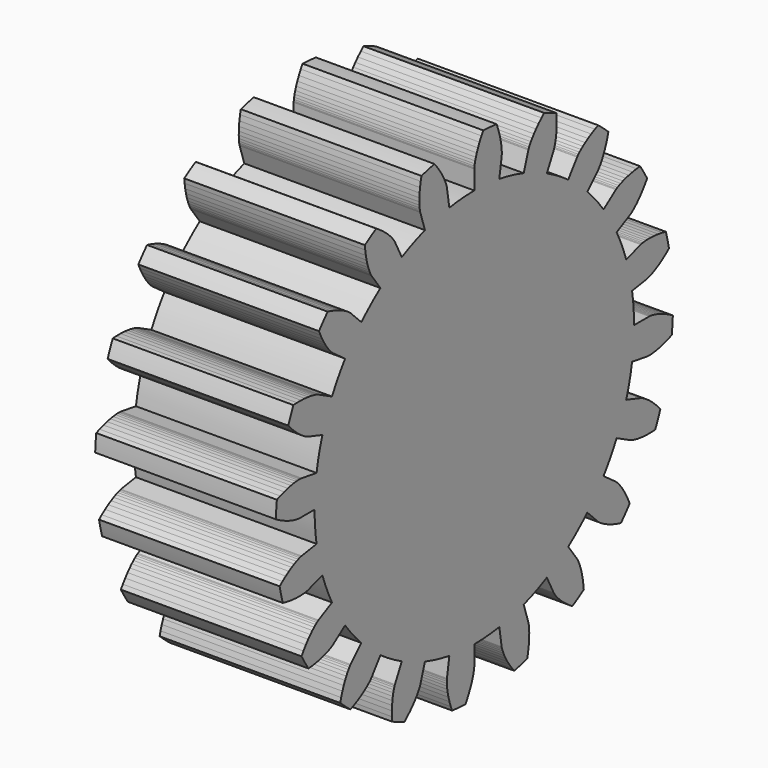
from build123d import *

# Parameters (mm, degrees)
F2_DEPTH = 12.7


# Not quite as in the source:
# - a variable given as a bare number and used for a length is read in inches; the dataset says mm whatever the document's units were


with BuildPart() as f2:
    # F1 (on Right) → F2 (new body)
    with BuildSketch(Plane.YZ):
        with BuildLine():
            ThreePointArc((13.8654281935, -2.1960680843), (13.9949872217, -1.1014293813), (14.0382625, 0))
            ThreePointArc((14.0382625, 0), (13.9949872217, 1.1014293813), (13.8654281935, 2.1960680843))
            ThreePointArc((13.8654281935, 2.1960680843), (13.6503841896, 3.2771672972), (13.3511810281, 4.338061684))
            ThreePointArc((13.3511810281, 4.338061684), (12.9696633958, 5.3722104779), (12.5081834758, 6.3732378078))
            ThreePointArc((12.5081834758, 6.3732378078), (11.9695864452, 7.3349720074), (11.357192934, 8.2514836653))
            ThreePointArc((11.357192934, 8.2514836653), (10.6747785517, 9.1171221826), (9.9265506098, 9.9265506098))
            ThreePointArc((9.9265506098, 9.9265506098), (9.1171221826, 10.6747785517), (8.2514836653, 11.357192934))
            ThreePointArc((8.2514836653, 11.357192934), (7.3349720074, 11.9695864452), (6.3732378078, 12.5081834758))
            ThreePointArc((6.3732378078, 12.5081834758), (5.3722104779, 12.9696633958), (4.338061684, 13.3511810281))
            ThreePointArc((4.338061684, 13.3511810281), (3.2771672972, 13.6503841896), (2.1960680843, 13.8654281935))
            ThreePointArc((2.1960680843, 13.8654281935), (1.1014293813, 13.9949872217), (0, 14.0382625))
            ThreePointArc((0, 14.0382625), (-1.1014293813, 13.9949872217), (-2.1960680843, 13.8654281935))
            ThreePointArc((-2.1960680843, 13.8654281935), (-3.2771672972, 13.6503841896), (-4.338061684, 13.3511810281))
            ThreePointArc((-4.338061684, 13.3511810281), (-5.3722104779, 12.9696633958), (-6.3732378078, 12.5081834758))
            ThreePointArc((-6.3732378078, 12.5081834758), (-7.3349720074, 11.9695864452), (-8.2514836653, 11.357192934))
            ThreePointArc((-8.2514836653, 11.357192934), (-9.1171221826, 10.6747785517), (-9.9265506098, 9.9265506098))
            ThreePointArc((-9.9265506098, 9.9265506098), (-10.6747785517, 9.1171221826), (-11.357192934, 8.2514836653))
            ThreePointArc((-11.357192934, 8.2514836653), (-11.9695864452, 7.3349720074), (-12.5081834758, 6.3732378078))
            ThreePointArc((-12.5081834758, 6.3732378078), (-12.9696633958, 5.3722104779), (-13.3511810281, 4.338061684))
            ThreePointArc((-13.3511810281, 4.338061684), (-13.6503841896, 3.2771672972), (-13.8654281935, 2.1960680843))
            ThreePointArc((-13.8654281935, 2.1960680843), (-13.9949872217, 1.1014293813), (-14.0382625, 0))
            ThreePointArc((-14.0382625, 0), (-13.9949872217, -1.1014293813), (-13.8654281935, -2.1960680843))
            ThreePointArc((-13.8654281935, -2.1960680843), (-13.6503841896, -3.2771672972), (-13.3511810281, -4.338061684))
            ThreePointArc((-13.3511810281, -4.338061684), (-12.9696633958, -5.3722104779), (-12.5081834758, -6.3732378078))
            ThreePointArc((-12.5081834758, -6.3732378078), (-11.9695864452, -7.3349720074), (-11.357192934, -8.2514836653))
            ThreePointArc((-11.357192934, -8.2514836653), (-10.6747785517, -9.1171221826), (-9.9265506098, -9.9265506098))
            ThreePointArc((-9.9265506098, -9.9265506098), (-9.1171221826, -10.6747785517), (-8.2514836653, -11.357192934))
            ThreePointArc((-8.2514836653, -11.357192934), (-7.3349720074, -11.9695864452), (-6.3732378078, -12.5081834758))
            ThreePointArc((-6.3732378078, -12.5081834758), (-5.3722104779, -12.9696633958), (-4.338061684, -13.3511810281))
            ThreePointArc((-4.338061684, -13.3511810281), (-3.2771672972, -13.6503841896), (-2.1960680843, -13.8654281935))
            ThreePointArc((-2.1960680843, -13.8654281935), (-1.1014293813, -13.9949872217), (0, -14.0382625))
            ThreePointArc((0, -14.0382625), (1.1014293813, -13.9949872217), (2.1960680843, -13.8654281935))
            ThreePointArc((2.1960680843, -13.8654281935), (3.2771672972, -13.6503841896), (4.338061684, -13.3511810281))
            ThreePointArc((4.338061684, -13.3511810281), (5.3722104779, -12.9696633958), (6.3732378078, -12.5081834758))
            ThreePointArc((6.3732378078, -12.5081834758), (7.3349720074, -11.9695864452), (8.2514836653, -11.357192934))
            ThreePointArc((8.2514836653, -11.357192934), (9.1171221826, -10.6747785517), (9.9265506098, -9.9265506098))
            ThreePointArc((9.9265506098, -9.9265506098), (10.6747785517, -9.1171221826), (11.357192934, -8.2514836653))
            ThreePointArc((11.357192934, -8.2514836653), (11.9695864452, -7.3349720074), (12.5081834758, -6.3732378078))
            ThreePointArc((12.5081834758, -6.3732378078), (12.9696633958, -5.3722104779), (13.3511810281, -4.338061684))
            ThreePointArc((13.3511810281, -4.338061684), (13.6503841896, -3.2771672972), (13.8654281935, -2.1960680843))
        make_face()
        with BuildLine():
            Line((-14.6171145636, -4.7493884238), (-13.3511810281, -4.338061684))
            ThreePointArc((-13.3511810281, -4.338061684), (-13.6503841896, -3.2771672972), (-13.8654281935, -2.1960680843))
            Line((-13.8654281935, -2.1960680843), (-15.180121665, -2.404295074))
            Line((-15.180121665, -2.404295074), (-15.1989848071, -2.4079309004))
            Line((-15.1989848071, -2.4079309004), (-15.2550320002, -2.4213414721))
            Line((-15.2550320002, -2.4213414721), (-15.3472398712, -2.4482306459))
            Line((-15.3472398712, -2.4482306459), (-15.474308977, -2.4922197725))
            Line((-15.474308977, -2.4922197725), (-15.6346697243, -2.5568294258))
            Line((-15.6346697243, -2.5568294258), (-15.8264894224, -2.6454615286))
            Line((-15.8264894224, -2.6454615286), (-16.0476804424, -2.7613819428))
            Line((-16.0476804424, -2.7613819428), (-16.2959094551, -2.9077035901))
            Line((-16.2959094551, -2.9077035901), (-16.5686077133, -3.0873701663))
            Line((-16.5686077133, -3.0873701663), (-16.8629823421, -3.3031405114))
            Line((-16.8629823421, -3.3031405114), (-17.1077308908, -3.5020636798))
            ThreePointArc((-17.1077308908, -3.5020636798), (-16.9800097349, -4.0765396663), (-16.8330034779, -4.6463857097))
            Line((-16.8330034779, -4.6463857097), (-16.5246216956, -4.7125140346))
            Line((-16.5246216956, -4.7125140346), (-16.1643742939, -4.771123535))
            Line((-16.1643742939, -4.771123535), (-15.8398314481, -4.807405208))
            Line((-15.8398314481, -4.807405208), (-15.5522291405, -4.8250851369))
            Line((-15.5522291405, -4.8250851369), (-15.3025197318, -4.8279523605))
            Line((-15.3025197318, -4.8279523605), (-15.0913689967, -4.8198398218))
            Line((-15.0913689967, -4.8198398218), (-14.9191543558, -4.8046051886))
            Line((-14.9191543558, -4.8046051886), (-14.7859643079, -4.7861116205))
            Line((-14.7859643079, -4.7861116205), (-14.6915990638, -4.7682085524))
            Line((-14.6915990638, -4.7682085524), (-14.635572377, -4.754712566))
            Line((-14.635572377, -4.754712566), (-14.6171145636, -4.7493884238))
        make_face()
        with BuildLine():
            Line((-12.4340603193, -9.0338736178), (-11.357192934, -8.2514836653))
            ThreePointArc((-11.357192934, -8.2514836653), (-11.9695864452, -7.3349720074), (-12.5081834758, -6.3732378078))
            Line((-12.5081834758, -6.3732378078), (-13.6941855903, -6.9775360683))
            Line((-13.6941855903, -6.9775360683), (-13.7110019723, -6.9868229763))
            Line((-13.7110019723, -6.9868229763), (-13.760161926, -7.016896723))
            Line((-13.760161926, -7.016896723), (-13.8395476109, -7.0709636461))
            Line((-13.8395476109, -7.0709636461), (-13.9468041243, -7.1520663048))
            Line((-13.9468041243, -7.1520663048), (-14.0793507771, -7.2630679327))
            Line((-14.0793507771, -7.2630679327), (-14.234393325, -7.4066376182))
            Line((-14.234393325, -7.4066376182), (-14.4089371079, -7.5852362677))
            Line((-14.4089371079, -7.5852362677), (-14.5998010523, -7.8011034073))
            Line((-14.5998010523, -7.8011034073), (-14.8036324824, -8.0562448714))
            Line((-14.8036324824, -8.0562448714), (-15.0169226878, -8.3524214272))
            Line((-15.0169226878, -8.3524214272), (-15.1882217503, -8.6172400636))
            ThreePointArc((-15.1882217503, -8.6172400636), (-14.88922887, -9.1241311864), (-14.5733254998, -9.6206595475))
            Line((-14.5733254998, -9.6206595475), (-14.25960222, -9.5882561103))
            Line((-14.25960222, -9.5882561103), (-13.8988752495, -9.5326744883))
            Line((-13.8988752495, -9.5326744883), (-13.5790050076, -9.466891155))
            Line((-13.5790050076, -9.466891155), (-13.3000155603, -9.3948317659))
            Line((-13.3000155603, -9.3948317659), (-13.0616417792, -9.3203942067))
            Line((-13.0616417792, -9.3203942067), (-12.863332409, -9.2474295583))
            Line((-12.863332409, -9.2474295583), (-12.7042543131, -9.1797233104))
            Line((-12.7042543131, -9.1797233104), (-12.583297877, -9.1209768938))
            Line((-12.583297877, -9.1209768938), (-12.4990835491, -9.0747896001))
            Line((-12.4990835491, -9.0747896001), (-12.4499694926, -9.0446409559))
            Line((-12.4499694926, -9.0446409559), (-12.4340603193, -9.0338736178))
        make_face()
        with BuildLine():
            Line((-9.0338736178, -12.4340603193), (-8.2514836653, -11.357192934))
            ThreePointArc((-8.2514836653, -11.357192934), (-9.1171221826, -10.6747785517), (-9.9265506098, -9.9265506098))
            Line((-9.9265506098, -9.9265506098), (-10.867767217, -10.867767217))
            Line((-10.867767217, -10.867767217), (-10.8808907344, -10.8817961392))
            Line((-10.8808907344, -10.8817961392), (-10.9183513298, -10.9255892331))
            Line((-10.9183513298, -10.9255892331), (-10.9771440047, -11.0015414583))
            Line((-10.9771440047, -11.0015414583), (-11.0540889108, -11.1118187557))
            Line((-11.0540889108, -11.1118187557), (-11.1458468793, -11.2583467456))
            Line((-11.1458468793, -11.2583467456), (-11.248935632, -11.4428004126))
            Line((-11.248935632, -11.4428004126), (-11.3597466163, -11.6665948172))
            Line((-11.3597466163, -11.6665948172), (-11.4745623996, -11.9308768694))
            Line((-11.4745623996, -11.9308768694), (-11.5895745611, -12.2365181973))
            Line((-11.5895745611, -12.2365181973), (-11.7009020117, -12.5841091389))
            Line((-11.7009020117, -12.5841091389), (-11.7819836423, -12.8889009502))
            ThreePointArc((-11.7819836423, -12.8889009502), (-11.340986544, -13.2785891743), (-10.8871088834, -13.6531961976))
            Line((-10.8871088834, -13.6531961976), (-10.5987535266, -13.5254328726))
            Line((-10.5987535266, -13.5254328726), (-10.2728574565, -13.3611008446))
            Line((-10.2728574565, -13.3611008446), (-9.9889709465, -13.1996918361))
            Line((-9.9889709465, -13.1996918361), (-9.7459037905, -13.0449468041))
            Line((-9.7459037905, -13.0449468041), (-9.5421993235, -12.900490929))
            Line((-9.5421993235, -12.900490929), (-9.3761432211, -12.7698164591))
            Line((-9.3761432211, -12.7698164591), (-9.2457733426, -12.6562661558))
            Line((-9.2457733426, -12.6562661558), (-9.1488905769, -12.5630173991))
            Line((-9.1488905769, -12.5630173991), (-9.0830706503, -12.4930670139))
            Line((-9.0830706503, -12.4930670139), (-9.0456768502, -12.4492168713))
            Line((-9.0456768502, -12.4492168713), (-9.0338736178, -12.4340603193))
        make_face()
        with BuildLine():
            Line((-4.7493884238, -14.6171145636), (-4.338061684, -13.3511810281))
            ThreePointArc((-4.338061684, -13.3511810281), (-5.3722104779, -12.9696633958), (-6.3732378078, -12.5081834758))
            Line((-6.3732378078, -12.5081834758), (-6.9775360683, -13.6941855903))
            Line((-6.9775360683, -13.6941855903), (-6.9856820997, -13.711583278))
            Line((-6.9856820997, -13.711583278), (-7.0077764328, -13.764808946))
            Line((-7.0077764328, -13.764808946), (-7.040221061, -13.8552117404))
            Line((-7.040221061, -13.8552117404), (-7.0793224564, -13.9838689663))
            Line((-7.0793224564, -13.9838689663), (-7.1213098312, -14.1515801375))
            Line((-7.1213098312, -14.1515801375), (-7.1623537435, -14.358862176))
            Line((-7.1623537435, -14.358862176), (-7.1985849778, -14.6059457801))
            Line((-7.1985849778, -14.6059457801), (-7.2261136314, -14.8927729763))
            Line((-7.2261136314, -14.8927729763), (-7.2410483324, -15.2189958653))
            Line((-7.2410483324, -15.2189958653), (-7.2395155218, -15.5839765695))
            Line((-7.2395155218, -15.5839765695), (-7.2224428854, -15.8989064095))
            ThreePointArc((-7.2224428854, -15.8989064095), (-6.6826094377, -16.1332463365), (-6.1351861945, -16.3492628766))
            Line((-6.1351861945, -16.3492628766), (-5.9004249921, -16.1386460281))
            Line((-5.9004249921, -16.1386460281), (-5.6412608004, -15.881649558))
            Line((-5.6412608004, -15.881649558), (-5.4211468118, -15.6404147126))
            Line((-5.4211468118, -15.6404147126), (-5.237795054, -15.4181315596))
            Line((-5.237795054, -15.4181315596), (-5.0886999135, -15.2177977161))
            Line((-5.0886999135, -15.2177977161), (-4.9711518072, -15.0422047523))
            Line((-4.9711518072, -15.0422047523), (-4.8822516582, -14.8939254884))
            Line((-4.8822516582, -14.8939254884), (-4.8189261231, -14.7753022297))
            Line((-4.8189261231, -14.7753022297), (-4.7779435107, -14.6884359841))
            Line((-4.7779435107, -14.6884359841), (-4.7559303328, -14.6351767006))
            Line((-4.7559303328, -14.6351767006), (-4.7493884238, -14.6171145636))
        make_face()
        with BuildLine():
            Line((0, -15.369343791), (0, -14.0382625))
            ThreePointArc((0, -14.0382625), (-1.1014293813, -13.9949872217), (-2.1960680843, -13.8654281935))
            Line((-2.1960680843, -13.8654281935), (-2.404295074, -15.180121665))
            Line((-2.404295074, -15.180121665), (-2.406666229, -15.1991851114))
            Line((-2.406666229, -15.1991851114), (-2.4112315526, -15.2566332542))
            Line((-2.4112315526, -15.2566332542), (-2.4141522278, -15.3526373623))
            Line((-2.4141522278, -15.3526373623), (-2.4115825954, -15.4870806511))
            Line((-2.4115825954, -15.4870806511), (-2.3996893598, -15.6595582657))
            Line((-2.3996893598, -15.6595582657), (-2.3746707675, -15.8693784656))
            Line((-2.3746707675, -15.8693784656), (-2.3327756863, -16.1155650045))
            Line((-2.3327756863, -16.1155650045), (-2.2703225136, -16.3968607002))
            Line((-2.2703225136, -16.3968607002), (-2.1837178417, -16.711732181))
            Line((-2.1837178417, -16.711732181), (-2.0694748119, -17.0583757934))
            Line((-2.0694748119, -17.0583757934), (-1.9559190973, -17.3526161352))
            ThreePointArc((-1.9559190973, -17.3526161352), (-1.3700919591, -17.4086689403), (-0.7827087346, -17.4449497932))
            Line((-0.7827087346, -17.4449497932), (-0.6245217488, -17.1720960658))
            Line((-0.6245217488, -17.1720960658), (-0.4574582322, -16.8475917587))
            Line((-0.4574582322, -16.8475917587), (-0.3226630559, -16.5501448238))
            Line((-0.3226630559, -16.5501448238), (-0.2169744437, -16.2820821735))
            Line((-0.2169744437, -16.2820821735), (-0.137083101, -16.0454804341))
            Line((-0.137083101, -16.0454804341), (-0.0795494184, -15.8421572392))
            Line((-0.0795494184, -15.8421572392), (-0.0408211648, -15.6736636222))
            Line((-0.0408211648, -15.6736636222), (-0.0172516049, -15.5412775325))
            Line((-0.0172516049, -15.5412775325), (-0.0051179705, -15.4459984999))
            Line((-0.0051179705, -15.4459984999), (-0.0006402179, -15.3885434651))
            Line((-0.0006402179, -15.3885434651), (0, -15.369343791))
        make_face()
        with BuildLine():
            Line((4.7493884238, -14.6171145636), (4.338061684, -13.3511810281))
            ThreePointArc((4.338061684, -13.3511810281), (3.2771672972, -13.6503841896), (2.1960680843, -13.8654281935))
            Line((2.1960680843, -13.8654281935), (2.404295074, -15.180121665))
            Line((2.404295074, -15.180121665), (2.4079309004, -15.1989848071))
            Line((2.4079309004, -15.1989848071), (2.4213414721, -15.2550320002))
            Line((2.4213414721, -15.2550320002), (2.4482306459, -15.3472398712))
            Line((2.4482306459, -15.3472398712), (2.4922197725, -15.474308977))
            Line((2.4922197725, -15.474308977), (2.5568294258, -15.6346697243))
            Line((2.5568294258, -15.6346697243), (2.6454615286, -15.8264894224))
            Line((2.6454615286, -15.8264894224), (2.7613819428, -16.0476804424))
            Line((2.7613819428, -16.0476804424), (2.9077035901, -16.2959094551))
            Line((2.9077035901, -16.2959094551), (3.0873701663, -16.5686077133))
            Line((3.0873701663, -16.5686077133), (3.3031405114, -16.8629823421))
            Line((3.3031405114, -16.8629823421), (3.5020636798, -17.1077308908))
            ThreePointArc((3.5020636798, -17.1077308908), (4.0765396663, -16.9800097349), (4.6463857097, -16.8330034779))
            Line((4.6463857097, -16.8330034779), (4.7125140346, -16.5246216956))
            Line((4.7125140346, -16.5246216956), (4.771123535, -16.1643742939))
            Line((4.771123535, -16.1643742939), (4.807405208, -15.8398314481))
            Line((4.807405208, -15.8398314481), (4.8250851369, -15.5522291405))
            Line((4.8250851369, -15.5522291405), (4.8279523605, -15.3025197318))
            Line((4.8279523605, -15.3025197318), (4.8198398218, -15.0913689967))
            Line((4.8198398218, -15.0913689967), (4.8046051886, -14.9191543558))
            Line((4.8046051886, -14.9191543558), (4.7861116205, -14.7859643079))
            Line((4.7861116205, -14.7859643079), (4.7682085524, -14.6915990638))
            Line((4.7682085524, -14.6915990638), (4.754712566, -14.635572377))
            Line((4.754712566, -14.635572377), (4.7493884238, -14.6171145636))
        make_face()
        with BuildLine():
            Line((9.0338736178, -12.4340603193), (8.2514836653, -11.357192934))
            ThreePointArc((8.2514836653, -11.357192934), (7.3349720074, -11.9695864452), (6.3732378078, -12.5081834758))
            Line((6.3732378078, -12.5081834758), (6.9775360683, -13.6941855903))
            Line((6.9775360683, -13.6941855903), (6.9868229763, -13.7110019723))
            Line((6.9868229763, -13.7110019723), (7.016896723, -13.760161926))
            Line((7.016896723, -13.760161926), (7.0709636461, -13.8395476109))
            Line((7.0709636461, -13.8395476109), (7.1520663048, -13.9468041243))
            Line((7.1520663048, -13.9468041243), (7.2630679327, -14.0793507771))
            Line((7.2630679327, -14.0793507771), (7.4066376182, -14.234393325))
            Line((7.4066376182, -14.234393325), (7.5852362677, -14.4089371079))
            Line((7.5852362677, -14.4089371079), (7.8011034073, -14.5998010523))
            Line((7.8011034073, -14.5998010523), (8.0562448714, -14.8036324824))
            Line((8.0562448714, -14.8036324824), (8.3524214272, -15.0169226878))
            Line((8.3524214272, -15.0169226878), (8.6172400636, -15.1882217503))
            ThreePointArc((8.6172400636, -15.1882217503), (9.1241311864, -14.88922887), (9.6206595475, -14.5733254998))
            Line((9.6206595475, -14.5733254998), (9.5882561103, -14.25960222))
            Line((9.5882561103, -14.25960222), (9.5326744883, -13.8988752495))
            Line((9.5326744883, -13.8988752495), (9.466891155, -13.5790050076))
            Line((9.466891155, -13.5790050076), (9.3948317659, -13.3000155603))
            Line((9.3948317659, -13.3000155603), (9.3203942067, -13.0616417792))
            Line((9.3203942067, -13.0616417792), (9.2474295583, -12.863332409))
            Line((9.2474295583, -12.863332409), (9.1797233104, -12.7042543131))
            Line((9.1797233104, -12.7042543131), (9.1209768938, -12.583297877))
            Line((9.1209768938, -12.583297877), (9.0747896001, -12.4990835491))
            Line((9.0747896001, -12.4990835491), (9.0446409559, -12.4499694926))
            Line((9.0446409559, -12.4499694926), (9.0338736178, -12.4340603193))
        make_face()
        with BuildLine():
            Line((12.4340603193, -9.0338736178), (11.357192934, -8.2514836653))
            ThreePointArc((11.357192934, -8.2514836653), (10.6747785517, -9.1171221826), (9.9265506098, -9.9265506098))
            Line((9.9265506098, -9.9265506098), (10.867767217, -10.867767217))
            Line((10.867767217, -10.867767217), (10.8817961392, -10.8808907344))
            Line((10.8817961392, -10.8808907344), (10.9255892331, -10.9183513298))
            Line((10.9255892331, -10.9183513298), (11.0015414583, -10.9771440047))
            Line((11.0015414583, -10.9771440047), (11.1118187557, -11.0540889108))
            Line((11.1118187557, -11.0540889108), (11.2583467456, -11.1458468793))
            Line((11.2583467456, -11.1458468793), (11.4428004126, -11.248935632))
            Line((11.4428004126, -11.248935632), (11.6665948172, -11.3597466163))
            Line((11.6665948172, -11.3597466163), (11.9308768694, -11.4745623996))
            Line((11.9308768694, -11.4745623996), (12.2365181973, -11.5895745611))
            Line((12.2365181973, -11.5895745611), (12.5841091389, -11.7009020117))
            Line((12.5841091389, -11.7009020117), (12.8889009502, -11.7819836423))
            ThreePointArc((12.8889009502, -11.7819836423), (13.2785891743, -11.340986544), (13.6531961976, -10.8871088834))
            Line((13.6531961976, -10.8871088834), (13.5254328726, -10.5987535266))
            Line((13.5254328726, -10.5987535266), (13.3611008446, -10.2728574565))
            Line((13.3611008446, -10.2728574565), (13.1996918361, -9.9889709465))
            Line((13.1996918361, -9.9889709465), (13.0449468041, -9.7459037905))
            Line((13.0449468041, -9.7459037905), (12.900490929, -9.5421993235))
            Line((12.900490929, -9.5421993235), (12.7698164591, -9.3761432211))
            Line((12.7698164591, -9.3761432211), (12.6562661558, -9.2457733426))
            Line((12.6562661558, -9.2457733426), (12.5630173991, -9.1488905769))
            Line((12.5630173991, -9.1488905769), (12.4930670139, -9.0830706503))
            Line((12.4930670139, -9.0830706503), (12.4492168713, -9.0456768502))
            Line((12.4492168713, -9.0456768502), (12.4340603193, -9.0338736178))
        make_face()
        with BuildLine():
            Line((14.6171145636, -4.7493884238), (13.3511810281, -4.338061684))
            ThreePointArc((13.3511810281, -4.338061684), (12.9696633958, -5.3722104779), (12.5081834758, -6.3732378078))
            Line((12.5081834758, -6.3732378078), (13.6941855903, -6.9775360683))
            Line((13.6941855903, -6.9775360683), (13.711583278, -6.9856820997))
            Line((13.711583278, -6.9856820997), (13.764808946, -7.0077764328))
            Line((13.764808946, -7.0077764328), (13.8552117404, -7.040221061))
            Line((13.8552117404, -7.040221061), (13.9838689663, -7.0793224564))
            Line((13.9838689663, -7.0793224564), (14.1515801375, -7.1213098312))
            Line((14.1515801375, -7.1213098312), (14.358862176, -7.1623537435))
            Line((14.358862176, -7.1623537435), (14.6059457801, -7.1985849778))
            Line((14.6059457801, -7.1985849778), (14.8927729763, -7.2261136314))
            Line((14.8927729763, -7.2261136314), (15.2189958653, -7.2410483324))
            Line((15.2189958653, -7.2410483324), (15.5839765695, -7.2395155218))
            Line((15.5839765695, -7.2395155218), (15.8989064095, -7.2224428854))
            ThreePointArc((15.8989064095, -7.2224428854), (16.1332463365, -6.6826094377), (16.3492628766, -6.1351861945))
            Line((16.3492628766, -6.1351861945), (16.1386460281, -5.9004249921))
            Line((16.1386460281, -5.9004249921), (15.881649558, -5.6412608004))
            Line((15.881649558, -5.6412608004), (15.6404147126, -5.4211468118))
            Line((15.6404147126, -5.4211468118), (15.4181315596, -5.237795054))
            Line((15.4181315596, -5.237795054), (15.2177977161, -5.0886999135))
            Line((15.2177977161, -5.0886999135), (15.0422047523, -4.9711518072))
            Line((15.0422047523, -4.9711518072), (14.8939254884, -4.8822516582))
            Line((14.8939254884, -4.8822516582), (14.7753022297, -4.8189261231))
            Line((14.7753022297, -4.8189261231), (14.6884359841, -4.7779435107))
            Line((14.6884359841, -4.7779435107), (14.6351767006, -4.7559303328))
            Line((14.6351767006, -4.7559303328), (14.6171145636, -4.7493884238))
        make_face()
        with BuildLine():
            Line((15.369343791, 0), (14.0382625, 0))
            ThreePointArc((14.0382625, 0), (13.9949872217, -1.1014293813), (13.8654281935, -2.1960680843))
            Line((13.8654281935, -2.1960680843), (15.180121665, -2.404295074))
            Line((15.180121665, -2.404295074), (15.1991851114, -2.406666229))
            Line((15.1991851114, -2.406666229), (15.2566332542, -2.4112315526))
            Line((15.2566332542, -2.4112315526), (15.3526373623, -2.4141522278))
            Line((15.3526373623, -2.4141522278), (15.4870806511, -2.4115825954))
            Line((15.4870806511, -2.4115825954), (15.6595582657, -2.3996893598))
            Line((15.6595582657, -2.3996893598), (15.8693784656, -2.3746707675))
            Line((15.8693784656, -2.3746707675), (16.1155650045, -2.3327756863))
            Line((16.1155650045, -2.3327756863), (16.3968607002, -2.2703225136))
            Line((16.3968607002, -2.2703225136), (16.711732181, -2.1837178417))
            Line((16.711732181, -2.1837178417), (17.0583757934, -2.0694748119))
            Line((17.0583757934, -2.0694748119), (17.3526161352, -1.9559190973))
            ThreePointArc((17.3526161352, -1.9559190973), (17.4086689403, -1.3700919591), (17.4449497932, -0.7827087346))
            Line((17.4449497932, -0.7827087346), (17.1720960658, -0.6245217488))
            Line((17.1720960658, -0.6245217488), (16.8475917587, -0.4574582322))
            Line((16.8475917587, -0.4574582322), (16.5501448238, -0.3226630559))
            Line((16.5501448238, -0.3226630559), (16.2820821735, -0.2169744437))
            Line((16.2820821735, -0.2169744437), (16.0454804341, -0.137083101))
            Line((16.0454804341, -0.137083101), (15.8421572392, -0.0795494184))
            Line((15.8421572392, -0.0795494184), (15.6736636222, -0.0408211648))
            Line((15.6736636222, -0.0408211648), (15.5412775325, -0.0172516049))
            Line((15.5412775325, -0.0172516049), (15.4459984999, -0.0051179705))
            Line((15.4459984999, -0.0051179705), (15.3885434651, -0.0006402179))
            Line((15.3885434651, -0.0006402179), (15.369343791, 0))
        make_face()
        with BuildLine():
            ThreePointArc((13.3511810281, 4.338061684), (13.6503841896, 3.2771672972), (13.8654281935, 2.1960680843))
            Line((13.8654281935, 2.1960680843), (15.180121665, 2.404295074))
            Line((15.180121665, 2.404295074), (15.1989848071, 2.4079309004))
            Line((15.1989848071, 2.4079309004), (15.2550320002, 2.4213414721))
            Line((15.2550320002, 2.4213414721), (15.3472398712, 2.4482306459))
            Line((15.3472398712, 2.4482306459), (15.474308977, 2.4922197725))
            Line((15.474308977, 2.4922197725), (15.6346697243, 2.5568294258))
            Line((15.6346697243, 2.5568294258), (15.8264894224, 2.6454615286))
            Line((15.8264894224, 2.6454615286), (16.0476804424, 2.7613819428))
            Line((16.0476804424, 2.7613819428), (16.2959094551, 2.9077035901))
            Line((16.2959094551, 2.9077035901), (16.5686077133, 3.0873701663))
            Line((16.5686077133, 3.0873701663), (16.8629823421, 3.3031405114))
            Line((16.8629823421, 3.3031405114), (17.1077308908, 3.5020636798))
            ThreePointArc((17.1077308908, 3.5020636798), (16.9800097349, 4.0765396663), (16.8330034779, 4.6463857097))
            Line((16.8330034779, 4.6463857097), (16.5246216956, 4.7125140346))
            Line((16.5246216956, 4.7125140346), (16.1643742939, 4.771123535))
            Line((16.1643742939, 4.771123535), (15.8398314481, 4.807405208))
            Line((15.8398314481, 4.807405208), (15.5522291405, 4.8250851369))
            Line((15.5522291405, 4.8250851369), (15.3025197318, 4.8279523605))
            Line((15.3025197318, 4.8279523605), (15.0913689967, 4.8198398218))
            Line((15.0913689967, 4.8198398218), (14.9191543558, 4.8046051886))
            Line((14.9191543558, 4.8046051886), (14.7859643079, 4.7861116205))
            Line((14.7859643079, 4.7861116205), (14.6915990638, 4.7682085524))
            Line((14.6915990638, 4.7682085524), (14.635572377, 4.754712566))
            Line((14.635572377, 4.754712566), (14.6171145636, 4.7493884238))
            Line((14.6171145636, 4.7493884238), (13.3511810281, 4.338061684))
        make_face()
        with BuildLine():
            ThreePointArc((11.357192934, 8.2514836653), (11.9695864452, 7.3349720074), (12.5081834758, 6.3732378078))
            Line((12.5081834758, 6.3732378078), (13.6941855903, 6.9775360683))
            Line((13.6941855903, 6.9775360683), (13.7110019723, 6.9868229763))
            Line((13.7110019723, 6.9868229763), (13.760161926, 7.016896723))
            Line((13.760161926, 7.016896723), (13.8395476109, 7.0709636461))
            Line((13.8395476109, 7.0709636461), (13.9468041243, 7.1520663048))
            Line((13.9468041243, 7.1520663048), (14.0793507771, 7.2630679327))
            Line((14.0793507771, 7.2630679327), (14.234393325, 7.4066376182))
            Line((14.234393325, 7.4066376182), (14.4089371079, 7.5852362677))
            Line((14.4089371079, 7.5852362677), (14.5998010523, 7.8011034073))
            Line((14.5998010523, 7.8011034073), (14.8036324824, 8.0562448714))
            Line((14.8036324824, 8.0562448714), (15.0169226878, 8.3524214272))
            Line((15.0169226878, 8.3524214272), (15.1882217503, 8.6172400636))
            ThreePointArc((15.1882217503, 8.6172400636), (14.88922887, 9.1241311864), (14.5733254998, 9.6206595475))
            Line((14.5733254998, 9.6206595475), (14.25960222, 9.5882561103))
            Line((14.25960222, 9.5882561103), (13.8988752495, 9.5326744883))
            Line((13.8988752495, 9.5326744883), (13.5790050076, 9.466891155))
            Line((13.5790050076, 9.466891155), (13.3000155603, 9.3948317659))
            Line((13.3000155603, 9.3948317659), (13.0616417792, 9.3203942067))
            Line((13.0616417792, 9.3203942067), (12.863332409, 9.2474295583))
            Line((12.863332409, 9.2474295583), (12.7042543131, 9.1797233104))
            Line((12.7042543131, 9.1797233104), (12.583297877, 9.1209768938))
            Line((12.583297877, 9.1209768938), (12.4990835491, 9.0747896001))
            Line((12.4990835491, 9.0747896001), (12.4499694926, 9.0446409559))
            Line((12.4499694926, 9.0446409559), (12.4340603193, 9.0338736178))
            Line((12.4340603193, 9.0338736178), (11.357192934, 8.2514836653))
        make_face()
        with BuildLine():
            ThreePointArc((8.2514836653, 11.357192934), (9.1171221826, 10.6747785517), (9.9265506098, 9.9265506098))
            Line((9.9265506098, 9.9265506098), (10.867767217, 10.867767217))
            Line((10.867767217, 10.867767217), (10.8808907344, 10.8817961392))
            Line((10.8808907344, 10.8817961392), (10.9183513298, 10.9255892331))
            Line((10.9183513298, 10.9255892331), (10.9771440047, 11.0015414583))
            Line((10.9771440047, 11.0015414583), (11.0540889108, 11.1118187557))
            Line((11.0540889108, 11.1118187557), (11.1458468793, 11.2583467456))
            Line((11.1458468793, 11.2583467456), (11.248935632, 11.4428004126))
            Line((11.248935632, 11.4428004126), (11.3597466163, 11.6665948172))
            Line((11.3597466163, 11.6665948172), (11.4745623996, 11.9308768694))
            Line((11.4745623996, 11.9308768694), (11.5895745611, 12.2365181973))
            Line((11.5895745611, 12.2365181973), (11.7009020117, 12.5841091389))
            Line((11.7009020117, 12.5841091389), (11.7819836423, 12.8889009502))
            ThreePointArc((11.7819836423, 12.8889009502), (11.340986544, 13.2785891743), (10.8871088834, 13.6531961976))
            Line((10.8871088834, 13.6531961976), (10.5987535266, 13.5254328726))
            Line((10.5987535266, 13.5254328726), (10.2728574565, 13.3611008446))
            Line((10.2728574565, 13.3611008446), (9.9889709465, 13.1996918361))
            Line((9.9889709465, 13.1996918361), (9.7459037905, 13.0449468041))
            Line((9.7459037905, 13.0449468041), (9.5421993235, 12.900490929))
            Line((9.5421993235, 12.900490929), (9.3761432211, 12.7698164591))
            Line((9.3761432211, 12.7698164591), (9.2457733426, 12.6562661558))
            Line((9.2457733426, 12.6562661558), (9.1488905769, 12.5630173991))
            Line((9.1488905769, 12.5630173991), (9.0830706503, 12.4930670139))
            Line((9.0830706503, 12.4930670139), (9.0456768502, 12.4492168713))
            Line((9.0456768502, 12.4492168713), (9.0338736178, 12.4340603193))
            Line((9.0338736178, 12.4340603193), (8.2514836653, 11.357192934))
        make_face()
        with BuildLine():
            ThreePointArc((4.338061684, 13.3511810281), (5.3722104779, 12.9696633958), (6.3732378078, 12.5081834758))
            Line((6.3732378078, 12.5081834758), (6.9775360683, 13.6941855903))
            Line((6.9775360683, 13.6941855903), (6.9856820997, 13.711583278))
            Line((6.9856820997, 13.711583278), (7.0077764328, 13.764808946))
            Line((7.0077764328, 13.764808946), (7.040221061, 13.8552117404))
            Line((7.040221061, 13.8552117404), (7.0793224564, 13.9838689663))
            Line((7.0793224564, 13.9838689663), (7.1213098312, 14.1515801375))
            Line((7.1213098312, 14.1515801375), (7.1623537435, 14.358862176))
            Line((7.1623537435, 14.358862176), (7.1985849778, 14.6059457801))
            Line((7.1985849778, 14.6059457801), (7.2261136314, 14.8927729763))
            Line((7.2261136314, 14.8927729763), (7.2410483324, 15.2189958653))
            Line((7.2410483324, 15.2189958653), (7.2395155218, 15.5839765695))
            Line((7.2395155218, 15.5839765695), (7.2224428854, 15.8989064095))
            ThreePointArc((7.2224428854, 15.8989064095), (6.6826094377, 16.1332463365), (6.1351861945, 16.3492628766))
            Line((6.1351861945, 16.3492628766), (5.9004249921, 16.1386460281))
            Line((5.9004249921, 16.1386460281), (5.6412608004, 15.881649558))
            Line((5.6412608004, 15.881649558), (5.4211468118, 15.6404147126))
            Line((5.4211468118, 15.6404147126), (5.237795054, 15.4181315596))
            Line((5.237795054, 15.4181315596), (5.0886999135, 15.2177977161))
            Line((5.0886999135, 15.2177977161), (4.9711518072, 15.0422047523))
            Line((4.9711518072, 15.0422047523), (4.8822516582, 14.8939254884))
            Line((4.8822516582, 14.8939254884), (4.8189261231, 14.7753022297))
            Line((4.8189261231, 14.7753022297), (4.7779435107, 14.6884359841))
            Line((4.7779435107, 14.6884359841), (4.7559303328, 14.6351767006))
            Line((4.7559303328, 14.6351767006), (4.7493884238, 14.6171145636))
            Line((4.7493884238, 14.6171145636), (4.338061684, 13.3511810281))
        make_face()
        with BuildLine():
            ThreePointArc((0, 14.0382625), (1.1014293813, 13.9949872217), (2.1960680843, 13.8654281935))
            Line((2.1960680843, 13.8654281935), (2.404295074, 15.180121665))
            Line((2.404295074, 15.180121665), (2.406666229, 15.1991851114))
            Line((2.406666229, 15.1991851114), (2.4112315526, 15.2566332542))
            Line((2.4112315526, 15.2566332542), (2.4141522278, 15.3526373623))
            Line((2.4141522278, 15.3526373623), (2.4115825954, 15.4870806511))
            Line((2.4115825954, 15.4870806511), (2.3996893598, 15.6595582657))
            Line((2.3996893598, 15.6595582657), (2.3746707675, 15.8693784656))
            Line((2.3746707675, 15.8693784656), (2.3327756863, 16.1155650045))
            Line((2.3327756863, 16.1155650045), (2.2703225136, 16.3968607002))
            Line((2.2703225136, 16.3968607002), (2.1837178417, 16.711732181))
            Line((2.1837178417, 16.711732181), (2.0694748119, 17.0583757934))
            Line((2.0694748119, 17.0583757934), (1.9559190973, 17.3526161352))
            ThreePointArc((1.9559190973, 17.3526161352), (1.3700919591, 17.4086689403), (0.7827087346, 17.4449497932))
            Line((0.7827087346, 17.4449497932), (0.6245217488, 17.1720960658))
            Line((0.6245217488, 17.1720960658), (0.4574582322, 16.8475917587))
            Line((0.4574582322, 16.8475917587), (0.3226630559, 16.5501448238))
            Line((0.3226630559, 16.5501448238), (0.2169744437, 16.2820821735))
            Line((0.2169744437, 16.2820821735), (0.137083101, 16.0454804341))
            Line((0.137083101, 16.0454804341), (0.0795494184, 15.8421572392))
            Line((0.0795494184, 15.8421572392), (0.0408211648, 15.6736636222))
            Line((0.0408211648, 15.6736636222), (0.0172516049, 15.5412775325))
            Line((0.0172516049, 15.5412775325), (0.0051179705, 15.4459984999))
            Line((0.0051179705, 15.4459984999), (0.0006402179, 15.3885434651))
            Line((0.0006402179, 15.3885434651), (0, 15.369343791))
            Line((0, 15.369343791), (0, 14.0382625))
        make_face()
        with BuildLine():
            ThreePointArc((-4.338061684, 13.3511810281), (-3.2771672972, 13.6503841896), (-2.1960680843, 13.8654281935))
            Line((-2.1960680843, 13.8654281935), (-2.404295074, 15.180121665))
            Line((-2.404295074, 15.180121665), (-2.4079309004, 15.1989848071))
            Line((-2.4079309004, 15.1989848071), (-2.4213414721, 15.2550320002))
            Line((-2.4213414721, 15.2550320002), (-2.4482306459, 15.3472398712))
            Line((-2.4482306459, 15.3472398712), (-2.4922197725, 15.474308977))
            Line((-2.4922197725, 15.474308977), (-2.5568294258, 15.6346697243))
            Line((-2.5568294258, 15.6346697243), (-2.6454615286, 15.8264894224))
            Line((-2.6454615286, 15.8264894224), (-2.7613819428, 16.0476804424))
            Line((-2.7613819428, 16.0476804424), (-2.9077035901, 16.2959094551))
            Line((-2.9077035901, 16.2959094551), (-3.0873701663, 16.5686077133))
            Line((-3.0873701663, 16.5686077133), (-3.3031405114, 16.8629823421))
            Line((-3.3031405114, 16.8629823421), (-3.5020636798, 17.1077308908))
            ThreePointArc((-3.5020636798, 17.1077308908), (-4.0765396663, 16.9800097349), (-4.6463857097, 16.8330034779))
            Line((-4.6463857097, 16.8330034779), (-4.7125140346, 16.5246216956))
            Line((-4.7125140346, 16.5246216956), (-4.771123535, 16.1643742939))
            Line((-4.771123535, 16.1643742939), (-4.807405208, 15.8398314481))
            Line((-4.807405208, 15.8398314481), (-4.8250851369, 15.5522291405))
            Line((-4.8250851369, 15.5522291405), (-4.8279523605, 15.3025197318))
            Line((-4.8279523605, 15.3025197318), (-4.8198398218, 15.0913689967))
            Line((-4.8198398218, 15.0913689967), (-4.8046051886, 14.9191543558))
            Line((-4.8046051886, 14.9191543558), (-4.7861116205, 14.7859643079))
            Line((-4.7861116205, 14.7859643079), (-4.7682085524, 14.6915990638))
            Line((-4.7682085524, 14.6915990638), (-4.754712566, 14.635572377))
            Line((-4.754712566, 14.635572377), (-4.7493884238, 14.6171145636))
            Line((-4.7493884238, 14.6171145636), (-4.338061684, 13.3511810281))
        make_face()
        with BuildLine():
            ThreePointArc((-8.2514836653, 11.357192934), (-7.3349720074, 11.9695864452), (-6.3732378078, 12.5081834758))
            Line((-6.3732378078, 12.5081834758), (-6.9775360683, 13.6941855903))
            Line((-6.9775360683, 13.6941855903), (-6.9868229763, 13.7110019723))
            Line((-6.9868229763, 13.7110019723), (-7.016896723, 13.760161926))
            Line((-7.016896723, 13.760161926), (-7.0709636461, 13.8395476109))
            Line((-7.0709636461, 13.8395476109), (-7.1520663048, 13.9468041243))
            Line((-7.1520663048, 13.9468041243), (-7.2630679327, 14.0793507771))
            Line((-7.2630679327, 14.0793507771), (-7.4066376182, 14.234393325))
            Line((-7.4066376182, 14.234393325), (-7.5852362677, 14.4089371079))
            Line((-7.5852362677, 14.4089371079), (-7.8011034073, 14.5998010523))
            Line((-7.8011034073, 14.5998010523), (-8.0562448714, 14.8036324824))
            Line((-8.0562448714, 14.8036324824), (-8.3524214272, 15.0169226878))
            Line((-8.3524214272, 15.0169226878), (-8.6172400636, 15.1882217503))
            ThreePointArc((-8.6172400636, 15.1882217503), (-9.1241311864, 14.88922887), (-9.6206595475, 14.5733254998))
            Line((-9.6206595475, 14.5733254998), (-9.5882561103, 14.25960222))
            Line((-9.5882561103, 14.25960222), (-9.5326744883, 13.8988752495))
            Line((-9.5326744883, 13.8988752495), (-9.466891155, 13.5790050076))
            Line((-9.466891155, 13.5790050076), (-9.3948317659, 13.3000155603))
            Line((-9.3948317659, 13.3000155603), (-9.3203942067, 13.0616417792))
            Line((-9.3203942067, 13.0616417792), (-9.2474295583, 12.863332409))
            Line((-9.2474295583, 12.863332409), (-9.1797233104, 12.7042543131))
            Line((-9.1797233104, 12.7042543131), (-9.1209768938, 12.583297877))
            Line((-9.1209768938, 12.583297877), (-9.0747896001, 12.4990835491))
            Line((-9.0747896001, 12.4990835491), (-9.0446409559, 12.4499694926))
            Line((-9.0446409559, 12.4499694926), (-9.0338736178, 12.4340603193))
            Line((-9.0338736178, 12.4340603193), (-8.2514836653, 11.357192934))
        make_face()
        with BuildLine():
            ThreePointArc((-11.357192934, 8.2514836653), (-10.6747785517, 9.1171221826), (-9.9265506098, 9.9265506098))
            Line((-9.9265506098, 9.9265506098), (-10.867767217, 10.867767217))
            Line((-10.867767217, 10.867767217), (-10.8817961392, 10.8808907344))
            Line((-10.8817961392, 10.8808907344), (-10.9255892331, 10.9183513298))
            Line((-10.9255892331, 10.9183513298), (-11.0015414583, 10.9771440047))
            Line((-11.0015414583, 10.9771440047), (-11.1118187557, 11.0540889108))
            Line((-11.1118187557, 11.0540889108), (-11.2583467456, 11.1458468793))
            Line((-11.2583467456, 11.1458468793), (-11.4428004126, 11.248935632))
            Line((-11.4428004126, 11.248935632), (-11.6665948172, 11.3597466163))
            Line((-11.6665948172, 11.3597466163), (-11.9308768694, 11.4745623996))
            Line((-11.9308768694, 11.4745623996), (-12.2365181973, 11.5895745611))
            Line((-12.2365181973, 11.5895745611), (-12.5841091389, 11.7009020117))
            Line((-12.5841091389, 11.7009020117), (-12.8889009502, 11.7819836423))
            ThreePointArc((-12.8889009502, 11.7819836423), (-13.2785891743, 11.340986544), (-13.6531961976, 10.8871088834))
            Line((-13.6531961976, 10.8871088834), (-13.5254328726, 10.5987535266))
            Line((-13.5254328726, 10.5987535266), (-13.3611008446, 10.2728574565))
            Line((-13.3611008446, 10.2728574565), (-13.1996918361, 9.9889709465))
            Line((-13.1996918361, 9.9889709465), (-13.0449468041, 9.7459037905))
            Line((-13.0449468041, 9.7459037905), (-12.900490929, 9.5421993235))
            Line((-12.900490929, 9.5421993235), (-12.7698164591, 9.3761432211))
            Line((-12.7698164591, 9.3761432211), (-12.6562661558, 9.2457733426))
            Line((-12.6562661558, 9.2457733426), (-12.5630173991, 9.1488905769))
            Line((-12.5630173991, 9.1488905769), (-12.4930670139, 9.0830706503))
            Line((-12.4930670139, 9.0830706503), (-12.4492168713, 9.0456768502))
            Line((-12.4492168713, 9.0456768502), (-12.4340603193, 9.0338736178))
            Line((-12.4340603193, 9.0338736178), (-11.357192934, 8.2514836653))
        make_face()
        with BuildLine():
            ThreePointArc((-13.3511810281, 4.338061684), (-12.9696633958, 5.3722104779), (-12.5081834758, 6.3732378078))
            Line((-12.5081834758, 6.3732378078), (-13.6941855903, 6.9775360683))
            Line((-13.6941855903, 6.9775360683), (-13.711583278, 6.9856820997))
            Line((-13.711583278, 6.9856820997), (-13.764808946, 7.0077764328))
            Line((-13.764808946, 7.0077764328), (-13.8552117404, 7.040221061))
            Line((-13.8552117404, 7.040221061), (-13.9838689663, 7.0793224564))
            Line((-13.9838689663, 7.0793224564), (-14.1515801375, 7.1213098312))
            Line((-14.1515801375, 7.1213098312), (-14.358862176, 7.1623537435))
            Line((-14.358862176, 7.1623537435), (-14.6059457801, 7.1985849778))
            Line((-14.6059457801, 7.1985849778), (-14.8927729763, 7.2261136314))
            Line((-14.8927729763, 7.2261136314), (-15.2189958653, 7.2410483324))
            Line((-15.2189958653, 7.2410483324), (-15.5839765695, 7.2395155218))
            Line((-15.5839765695, 7.2395155218), (-15.8989064095, 7.2224428854))
            ThreePointArc((-15.8989064095, 7.2224428854), (-16.1332463365, 6.6826094377), (-16.3492628766, 6.1351861945))
            Line((-16.3492628766, 6.1351861945), (-16.1386460281, 5.9004249921))
            Line((-16.1386460281, 5.9004249921), (-15.881649558, 5.6412608004))
            Line((-15.881649558, 5.6412608004), (-15.6404147126, 5.4211468118))
            Line((-15.6404147126, 5.4211468118), (-15.4181315596, 5.237795054))
            Line((-15.4181315596, 5.237795054), (-15.2177977161, 5.0886999135))
            Line((-15.2177977161, 5.0886999135), (-15.0422047523, 4.9711518072))
            Line((-15.0422047523, 4.9711518072), (-14.8939254884, 4.8822516582))
            Line((-14.8939254884, 4.8822516582), (-14.7753022297, 4.8189261231))
            Line((-14.7753022297, 4.8189261231), (-14.6884359841, 4.7779435107))
            Line((-14.6884359841, 4.7779435107), (-14.6351767006, 4.7559303328))
            Line((-14.6351767006, 4.7559303328), (-14.6171145636, 4.7493884238))
            Line((-14.6171145636, 4.7493884238), (-13.3511810281, 4.338061684))
        make_face()
        with BuildLine():
            ThreePointArc((-14.0382625, 0), (-13.9949872217, 1.1014293813), (-13.8654281935, 2.1960680843))
            Line((-13.8654281935, 2.1960680843), (-15.180121665, 2.404295074))
            Line((-15.180121665, 2.404295074), (-15.1991851114, 2.406666229))
            Line((-15.1991851114, 2.406666229), (-15.2566332542, 2.4112315526))
            Line((-15.2566332542, 2.4112315526), (-15.3526373623, 2.4141522278))
            Line((-15.3526373623, 2.4141522278), (-15.4870806511, 2.4115825954))
            Line((-15.4870806511, 2.4115825954), (-15.6595582657, 2.3996893598))
            Line((-15.6595582657, 2.3996893598), (-15.8693784656, 2.3746707675))
            Line((-15.8693784656, 2.3746707675), (-16.1155650045, 2.3327756863))
            Line((-16.1155650045, 2.3327756863), (-16.3968607002, 2.2703225136))
            Line((-16.3968607002, 2.2703225136), (-16.711732181, 2.1837178417))
            Line((-16.711732181, 2.1837178417), (-17.0583757934, 2.0694748119))
            Line((-17.0583757934, 2.0694748119), (-17.3526161352, 1.9559190973))
            ThreePointArc((-17.3526161352, 1.9559190973), (-17.4086689403, 1.3700919591), (-17.4449497932, 0.7827087346))
            Line((-17.4449497932, 0.7827087346), (-17.1720960658, 0.6245217488))
            Line((-17.1720960658, 0.6245217488), (-16.8475917587, 0.4574582322))
            Line((-16.8475917587, 0.4574582322), (-16.5501448238, 0.3226630559))
            Line((-16.5501448238, 0.3226630559), (-16.2820821735, 0.2169744437))
            Line((-16.2820821735, 0.2169744437), (-16.0454804341, 0.137083101))
            Line((-16.0454804341, 0.137083101), (-15.8421572392, 0.0795494184))
            Line((-15.8421572392, 0.0795494184), (-15.6736636222, 0.0408211648))
            Line((-15.6736636222, 0.0408211648), (-15.5412775325, 0.0172516049))
            Line((-15.5412775325, 0.0172516049), (-15.4459984999, 0.0051179705))
            Line((-15.4459984999, 0.0051179705), (-15.3885434651, 0.0006402179))
            Line((-15.3885434651, 0.0006402179), (-15.369343791, 0))
            Line((-15.369343791, 0), (-14.0382625, 0))
        make_face()
    extrude(amount=F2_DEPTH)


solid = f2.part
